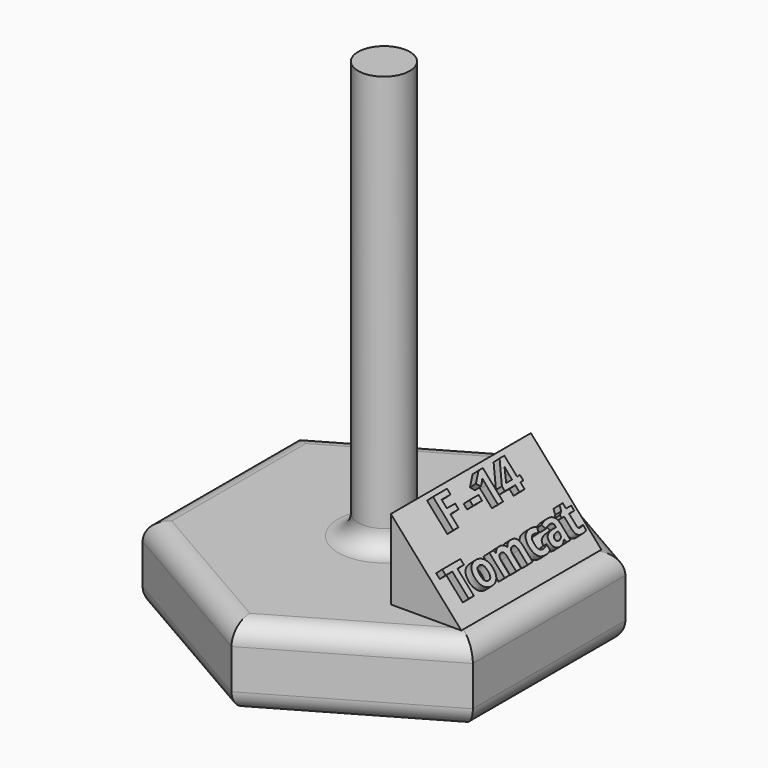
from build123d import *

# Parameters (mm, degrees)
F0_R         = 6.5
F1_DEPTH     = 20
F2_DEPTH     = 125
F3_R         = 5
F5_DEPTH     = 22
F6_TEXT_SIZE = 10.7700592353
F7_DEPTH     = 2
F8_TEXT_SIZE = 10.6237290949
F9_DEPTH     = 2


# Not quite as in the source:
# - Text() gives the source's letters only with a copy of the font that has no kerning and outlines rounded to 1/6400 em; it was checked with that copy


with BuildPart() as f1:
    # F0 (on Top) → F1 (new body)
    with BuildSketch(Plane.XY):
        Polygon((41.5, -23.9600361714), (41.5, 23.9600361714), (0, 47.9200723427), (-41.5, 23.9600361714), (-41.5, -23.9600361714), (0, -47.9200723427), align=None)
        Circle(F0_R, mode=Mode.SUBTRACT)
    extrude(amount=F1_DEPTH)

    # F0 (on Top) → F2 (join)
    with BuildSketch(Plane.XY):
        Circle(F0_R)
    extrude(amount=F2_DEPTH)

    # F3
    f3_edges = [f1.edges().sort_by_distance(p)[0] for p in [
        (41.5, 0, 20),
        (20.75, 35.940054, 20),
        (-20.75, 35.940054, 20),
        (-41.5, 0, 20),
        (-20.75, -35.940054, 20),
        (20.75, -35.940054, 20),
        (-6.5, 0, 20),
        (-20.75, 35.940054, 0),
        (-41.5, 0, 0),
        (41.5, 0, 0),
        (20.75, 35.940054, 0),
        (-20.75, -35.940054, 0),
        (20.75, -35.940054, 0),
    ]]
    fillet(f3_edges, radius=F3_R)


with BuildPart() as f5:
    # F4 (on Front) → F5 (new body, symmetric)
    with BuildSketch(Plane.XZ):
        Polygon((19.3288903683, 40.0872047422), (19.3288903683, 20.0498886406), (37.0393693447, 20.0498886406), align=None)
    extrude(amount=F5_DEPTH, both=True)

    # F6 (on face) → F7 (join)
    with BuildSketch(Plane(origin=(30.7432599733, 0, 27.1731930895), x_dir=(0, 1, 0), z_dir=(0.7492718712, 0, 0.6622625333))):
        with Locations((-12.6622533543, 8.2651593178)):
            Text('F -14', F6_TEXT_SIZE, font='Open Sans', font_style=FontStyle.BOLD, text_align=(TextAlign.LEFT, TextAlign.BOTTOM))
    extrude(amount=F7_DEPTH)

    # F8 (on face) → F9 (join)
    with BuildSketch(Plane(origin=(30.7432599733, 0, 27.1731930895), x_dir=(0, 1, 0), z_dir=(0.7492718712, 0, 0.6622625333))):
        with Locations((-20, -4.8890496019)):
            Text('Tomcat', F8_TEXT_SIZE, font='Open Sans', font_style=FontStyle.BOLD, text_align=(TextAlign.LEFT, TextAlign.BOTTOM))
    extrude(amount=F9_DEPTH)


solid = Compound([f1.part, f5.part])
